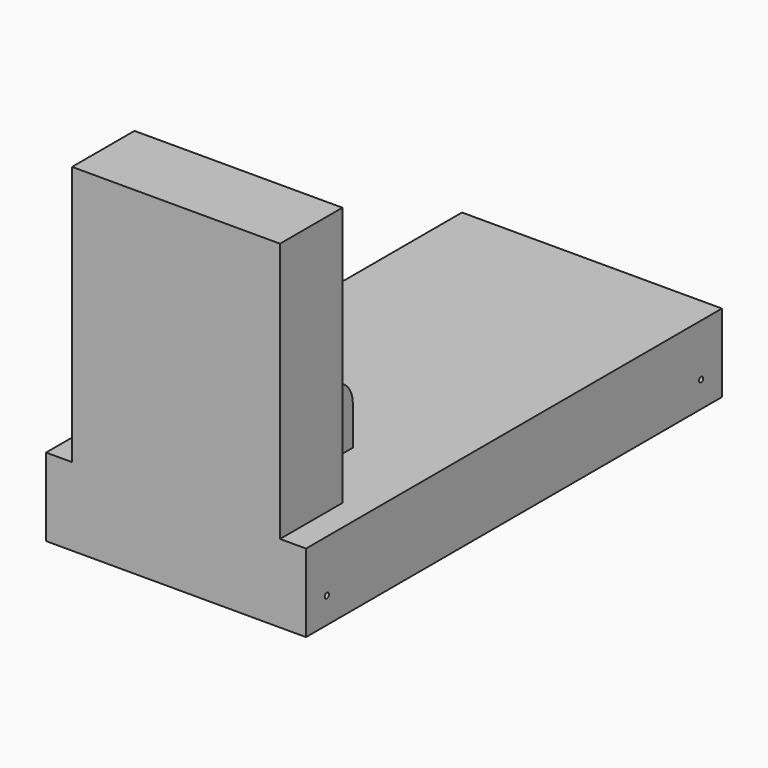
from build123d import *

# Parameters (mm, degrees)
F0_W      = 200
F0_H      = 30
F1_DEPTH  = 50
F2_W      = 80
F2_H      = 30
F3_DEPTH  = 100
F5_DEPTH  = 25
F6_R      = 3.75
F7_DEPTH  = 70.001
F8_R      = 9.99999
F9_R      = 1
F10_DEPTH = 100.001


# Not quite as in the source:
# - a fillet or chamfer is up to 0.001 mm smaller than in the source, because OpenCascade refuses the exact size


with BuildPart() as f1:
    # F0 (on Right) → F1 (new body, symmetric)
    with BuildSketch(Plane.YZ):
        Rectangle(F0_W, F0_H)
    extrude(amount=F1_DEPTH, both=True)

    # F2 (on face) → F3 (join)
    with BuildSketch(Plane.XY.offset(15)):
        with Locations((0, -85)):
            Rectangle(F2_W, F2_H)
    extrude(amount=F3_DEPTH)

    # F4 (on face) → F5 (join)
    with BuildSketch(Plane.XY.offset(15)):
        Polygon((-20, -40), (-20, -60), (0, -60), (20, -60), (20, -40), align=None)
    extrude(amount=F5_DEPTH)

    # F6 (on face) → F7 (cut, through all)
    with BuildSketch(Plane.YZ.offset(20)):
        with Locations((-50, 30)):
            Circle(F6_R)
    extrude(amount=-F7_DEPTH, mode=Mode.SUBTRACT)

    # F8 (radius 10 in the source; OpenCascade refuses exactly that, so slightly less here)
    f8_edges = [f1.edges().sort_by_distance(p)[0] for p in [
        (0, -40, 40),
        (0, -60, 40),
    ]]
    fillet(f8_edges, radius=F8_R)

    # F9 (on face) → F10 (cut, through all)
    with BuildSketch(Plane.YZ.offset(50)):
        with Locations((90, -5)):
            Circle(F9_R)
        with Locations((-90, -5)):
            Circle(F9_R)
    extrude(amount=-F10_DEPTH, mode=Mode.SUBTRACT)


solid = f1.part
